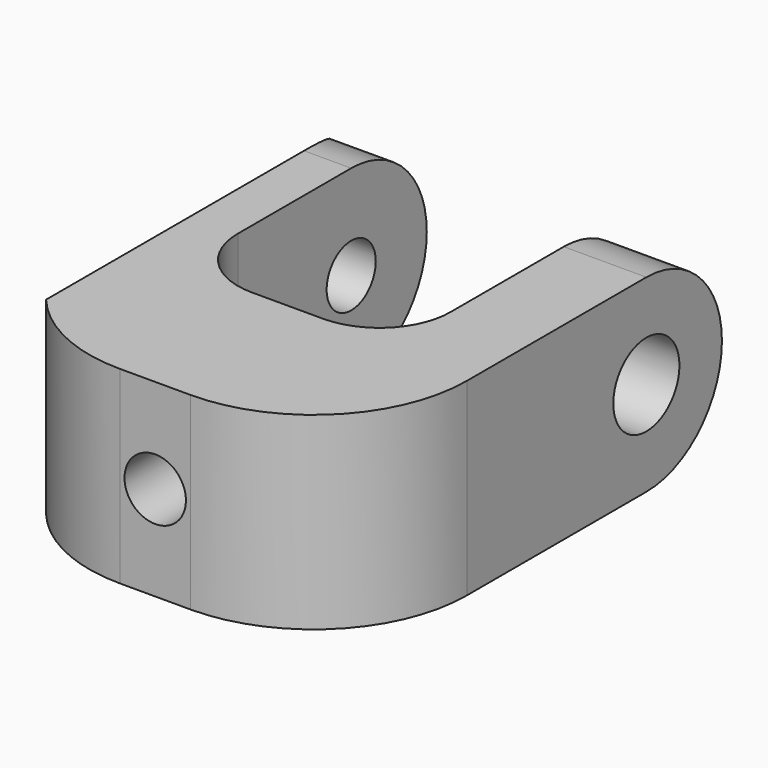
from build123d import *

# Parameters (mm, degrees)
F1_DEPTH    = 8
F3_DEPTH    = 16.001
F2_R        = 1.3
F4_DEPTH    = 16.001
F2_R_2      = 1.75
F5_DEPTH    = 3.5
F6_R        = 1.3
F7_DEPTH    = 7
F8_T1_DEPTH = 19.9153161013


# Not quite as in the source:
# - a fillet or chamfer that OpenCascade refuses, or shapes differently, is made with other operations: its cross-section is extruded or revolved along the edge and cut away or added


with BuildPart() as f1:
    # F0 (on Top) → F1 (new body)
    with BuildSketch(Plane.XY):
        with BuildLine():
            Line((-4.5, 3), (-4.5, 13))
            Line((-4.5, 13), (-8, 13))
            Line((-8, 13), (-8, -0.5))
            ThreePointArc((-8, -0.5), (-6.0961940777, -5.0961940777), (-1.5, -7))
            Line((-1.5, -7), (1.5, -7))
            ThreePointArc((1.5, -7), (6.0961940777, -5.0961940777), (8, -0.5))
            Line((8, -0.5), (8, 13))
            Line((8, 13), (4.5, 13))
            Line((4.5, 13), (4.5, 3))
            ThreePointArc((4.5, 3), (3.6213203436, 0.8786796564), (1.5, 0))
            Line((1.5, 0), (-1.5, 0))
            ThreePointArc((-1.5, 0), (-3.6213203436, 0.8786796564), (-4.5, 3))
        make_face()
    extrude(amount=F1_DEPTH)

    # F2 (on face) → F3 (cut, through all)
    with BuildSketch(Plane.YZ.offset(8)):
        with BuildLine():
            ThreePointArc((13, 4), (11.8284271247, 1.1715728753), (9, 0))
            Line((9, 0), (13, 0))
            Line((13, 0), (13, 4))
        make_face()
        with BuildLine():
            ThreePointArc((9, 8), (11.8284271247, 6.8284271247), (13, 4))
            Line((13, 4), (13, 8))
            Line((13, 8), (9, 8))
        make_face()
    extrude(amount=-F3_DEPTH, mode=Mode.SUBTRACT)

    # F2 (on face) → F4 (cut, through all)
    with BuildSketch(Plane.YZ.offset(8)):
        with Locations((9, 4)):
            Circle(F2_R)
    extrude(amount=-F4_DEPTH, mode=Mode.SUBTRACT)

    # F2 (on face) → F5 (cut, through all)
    with BuildSketch(Plane.YZ.offset(8)):
        with Locations((9, 4)):
            Circle(F2_R_2)
        with Locations((9, 4)):
            Circle(F2_R, mode=Mode.SUBTRACT)
    extrude(amount=-F5_DEPTH, mode=Mode.SUBTRACT)

    # F6 (on face) → F7 (cut, through all)
    with BuildSketch(Plane(origin=(0, 0, 0), x_dir=(-1, 0, 0), z_dir=(0, 1, 0))):
        with Locations((0, 4)):
            Circle(F6_R)
    extrude(amount=-F7_DEPTH, mode=Mode.SUBTRACT)

    # F8: chamfer of 1.5 on 2 edges, made by hand

    # F8_s2 → F8_t1 (cut)
    with BuildSketch(Plane.XZ.offset(-12.8575244819)):
        Polygon((-6.5, 0), (-8, 1.5), (-8, 0), align=None)
        Polygon((-6.5, 8), (-8, 6.5), (-8, 8), align=None)
    extrude(amount=F8_T1_DEPTH, mode=Mode.SUBTRACT)


solid = f1.part
